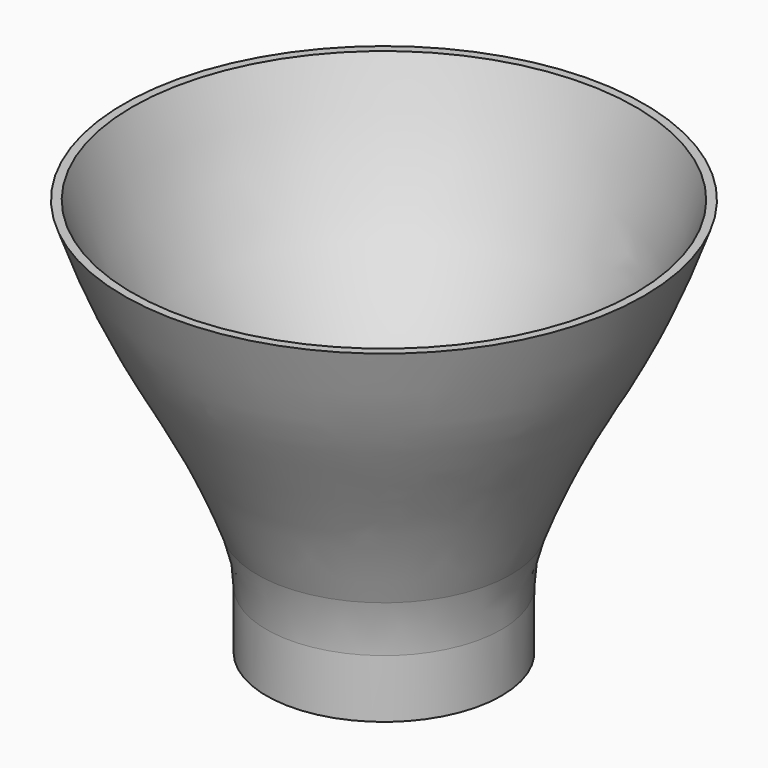
from build123d import *

# Parameters (mm, degrees)
F2_R     = 28
F2_R_2   = 26
F3_DEPTH = 20
F4_R     = 35


# Not quite as in the source:
# - a feature names something its author has since deleted; it is built from what else it names


with BuildPart() as f1:
    # F0 (on Front) → F1 (revolve)
    with BuildSketch(Plane.XZ):
        with BuildLine():
            add(Edge.make_bspline(
                [(26, -75), (32.5, -56.25), (43, -37.5), (53.5, -18.75), (60, 0)],
                knots=[0, 0, 0, 0, 0.5, 1, 1, 1, 1], degree=3))
            Line((26, -75), (28, -75))
            add(Edge.make_bspline(
                [(28, -75), (34.5, -56.25), (45, -37.5), (55.5, -18.75), (62, 0)],
                knots=[0, 0, 0, 0, 0.5, 1, 1, 1, 1], degree=3))
            Line((62, 0), (60, 0))
        make_face()
    revolve(axis=Axis((0, 0, -37.5), (0, 0, -1)))

    # F2 (on face) → F3 (join)
    with BuildSketch(Plane(origin=(0, 0, -75), x_dir=(1, 0, 0), z_dir=(0, 0, -1))):
        Circle(F2_R)
        Circle(F2_R_2, mode=Mode.SUBTRACT)
    extrude(amount=F3_DEPTH)

    # F4
    f4_edges = [f1.edges().sort_by_distance(p)[0] for p in [
        (-26, 0, -75),
        (-28, 0, -75),
    ]]
    fillet(f4_edges, radius=F4_R)


solid = f1.part
